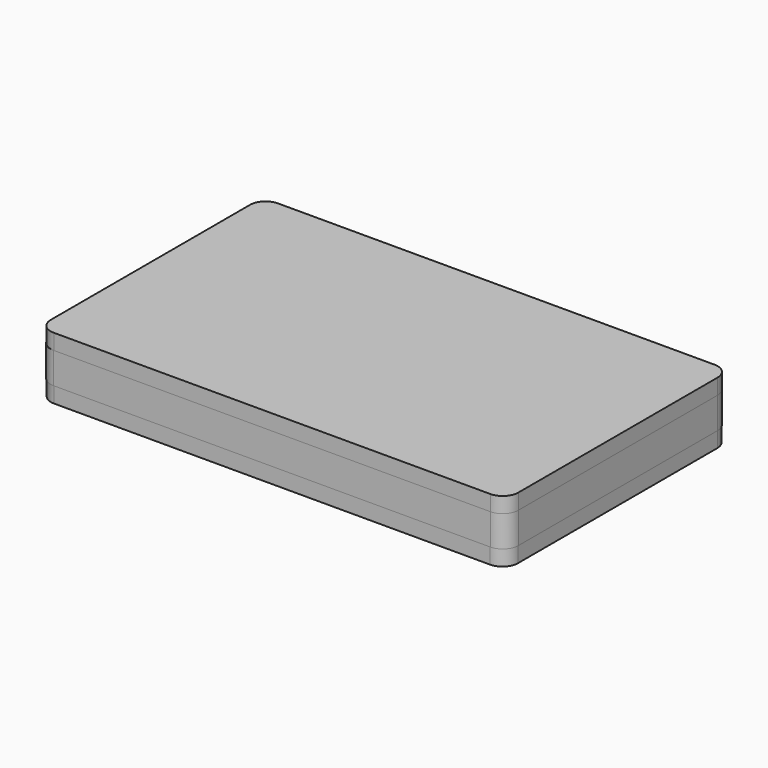
from build123d import *

# Parameters (mm, degrees)
F0_W           = 90.17
F0_H           = 52.07
F1_DEPTH       = 6.35
F2_W           = 95.377
F2_H           = 57.15
F2_W_2         = 90.17
F2_H_2         = 52.07
F3_DEPTH       = 3.175
F4_W           = 2.54
F4_H           = 12.7
F5_DEPTH       = 3.175
F8_DEPTH       = 6.35
F10_DEPTH      = 6.35
F11_R          = 1.9431941061
F12_F1_R       = 3.175
F12_F2_R       = 3.175
F12_F3_R       = 3.175
F12_F4_R       = 3.175
F12_2_F1_R     = 3.175
F12_2_F2_R     = 3.175
F12_2_F3_R     = 3.175
F12_2_F4_R     = 3.175
F12_3_T1_DEPTH = 21.9042598667
F12_3_T3_DEPTH = 22.225


# Not quite as in the source:
# - a fillet or chamfer that OpenCascade refuses, or shapes differently, is made with other operations: its cross-section is extruded or revolved along the edge and cut away or added


with BuildPart() as f1:
    # F0 (on Top) → F1 (new body)
    with BuildSketch(Plane.XY):
        Rectangle(F0_W, F0_H)
    extrude(amount=F1_DEPTH)


with BuildPart() as f3:
    # F2 (on face) → F3 (new body)
    with BuildSketch(Plane.XY.offset(6.35)):
        Rectangle(F2_W, F2_H)
        Rectangle(F2_W_2, F2_H_2, mode=Mode.SUBTRACT)
        Rectangle(F2_W_2, F2_H_2)
    extrude(amount=F3_DEPTH)

    # F12: fillet of radius 3.175 on 4 edges, made by hand

    # F12_f1
    f12_f1_edges = [f3.edges().sort_by_distance(p)[0] for p in [
        (47.6885, -28.575, 7.9375),
    ]]
    fillet(f12_f1_edges, radius=F12_F1_R)

    # F12_f2
    f12_f2_edges = [f3.edges().sort_by_distance(p)[0] for p in [
        (47.6885, 28.575, 7.9375),
    ]]
    fillet(f12_f2_edges, radius=F12_F2_R)

    # F12_f3
    f12_f3_edges = [f3.edges().sort_by_distance(p)[0] for p in [
        (-47.6885, 28.575, 7.9375),
    ]]
    fillet(f12_f3_edges, radius=F12_F3_R)

    # F12_f4
    f12_f4_edges = [f3.edges().sort_by_distance(p)[0] for p in [
        (-47.6885, -28.575, 7.9375),
    ]]
    fillet(f12_f4_edges, radius=F12_F4_R)


with BuildPart() as f5:
    # F4 (on face) → F5 (new body)
    with BuildSketch(Plane(origin=(0, 0, 0), x_dir=(1, 0, 0), z_dir=(0, 0, -1))):
        Polygon((47.625, 28.575), (-47.625, 28.575), (-47.625, 8.73125), (-45.085, 8.73125), (-45.085, 26.035), (45.085, 26.035), (45.085, -26.035), (-45.085, -26.035), (-45.085, -8.73125), (-47.625, -8.73125), (-47.625, -28.575), (47.625, -28.575), align=None)
        with BuildLine():
            Line((-45.085, 26.035), (-45.085, 8.73125))
            Line((-45.085, 8.73125), (15.2114481971, 8.73125))
            ThreePointArc((15.2114481971, 8.73125), (17.8489807487, 7.540625), (15.2114481971, 6.35))
            Line((15.2114481971, 6.35), (-45.085, 6.35))
            Line((-45.085, 6.35), (-45.085, -6.35))
            Line((-45.085, -6.35), (15.2114481971, -6.35))
            ThreePointArc((15.2114481971, -6.35), (17.8489807487, -7.540625), (15.2114481971, -8.73125))
            Line((15.2114481971, -8.73125), (-45.085, -8.73125))
            Line((-45.085, -8.73125), (-45.085, -26.035))
            Line((-45.085, -26.035), (45.085, -26.035))
            Line((45.085, -26.035), (45.085, 26.035))
            Line((45.085, 26.035), (-45.085, 26.035))
        make_face()
        with Locations((-46.355, 0)):
            Rectangle(F4_W, F4_H)
    extrude(amount=F5_DEPTH)

    # F12#2: fillet of radius 3.175 on 4 edges, made by hand

    # F12_2_f1
    f12_2_f1_edges = [f5.edges().sort_by_distance(p)[0] for p in [
        (47.625, -28.575, -1.5875),
    ]]
    fillet(f12_2_f1_edges, radius=F12_2_F1_R)

    # F12_2_f2
    f12_2_f2_edges = [f5.edges().sort_by_distance(p)[0] for p in [
        (-47.625, -28.575, -1.5875),
    ]]
    fillet(f12_2_f2_edges, radius=F12_2_F2_R)

    # F12_2_f3
    f12_2_f3_edges = [f5.edges().sort_by_distance(p)[0] for p in [
        (-47.625, 28.575, -1.5875),
    ]]
    fillet(f12_2_f3_edges, radius=F12_2_F3_R)

    # F12_2_f4
    f12_2_f4_edges = [f5.edges().sort_by_distance(p)[0] for p in [
        (47.625, 28.575, -1.5875),
    ]]
    fillet(f12_2_f4_edges, radius=F12_2_F4_R)


with BuildPart() as f8:
    # F7 (on face) → F8 (new body, through all)
    with BuildSketch(Plane(origin=(0, 0, 6.35), x_dir=(1, 0, 0), z_dir=(0, 0, -1))):
        Polygon((47.6885, 28.575), (-47.6885, 28.575), (-47.6885, 26.035), (-45.085, 26.035), (45.085, 26.035), (45.085, -26.035), (-45.085, -26.035), (-47.6885, -26.035), (-47.6885, -28.575), (47.6885, -28.575), align=None)
    extrude(amount=F8_DEPTH)

    # F12#3: fillet of radius 3.175 on 4 edges, made by hand

    # F12_3_s2 → F12_3_t1 (cut)
    with BuildSketch(Plane.XY.offset(-7.7771299333)):
        with BuildLine():
            ThreePointArc((-44.5776480267, -28.575), (-46.5856943409, -27.8593444248), (-47.6885, -26.035))
            Line((-47.6885, -26.035), (-47.6885, -28.575))
            Line((-47.6885, -28.575), (-44.5776480267, -28.575))
        make_face()
        with BuildLine():
            ThreePointArc((-44.5776480267, 28.575), (-46.5856943409, 27.8593444248), (-47.6885, 26.035))
            Line((-47.6885, 26.035), (-47.6885, 28.575))
            Line((-47.6885, 28.575), (-44.5776480267, 28.575))
        make_face()
    extrude(amount=F12_3_T1_DEPTH, mode=Mode.SUBTRACT)

    # F12_3_s4 → F12_3_t3 (cut)
    with BuildSketch(Plane.XY.offset(-7.9375)):
        with BuildLine():
            ThreePointArc((44.5135, -28.575), (46.7585640303, -27.6450640303), (47.6885, -25.4))
            Line((47.6885, -25.4), (47.6885, -28.575))
            Line((47.6885, -28.575), (44.5135, -28.575))
        make_face()
        with BuildLine():
            ThreePointArc((44.5135, 28.575), (46.7585640303, 27.6450640303), (47.6885, 25.4))
            Line((47.6885, 25.4), (47.6885, 28.575))
            Line((47.6885, 28.575), (44.5135, 28.575))
        make_face()
    extrude(amount=F12_3_T3_DEPTH, mode=Mode.SUBTRACT)


with BuildPart() as f10:
    # F9 (on Front) → F10 (new body, symmetric)
    with BuildSketch(Plane.XZ):
        Polygon((-42.4429178238, 5.3962194361), (-47.5056767464, 0), (-38.0619131029, 0), align=None)
    extrude(amount=F10_DEPTH, both=True)

    # F11
    f11_edges = [f10.edges().sort_by_distance(p)[0] for p in [
        (-42.442918, 0, 5.396219),
    ]]
    fillet(f11_edges, radius=F11_R)


solid = Compound([f1.part, f3.part, f5.part, f8.part, f10.part])
